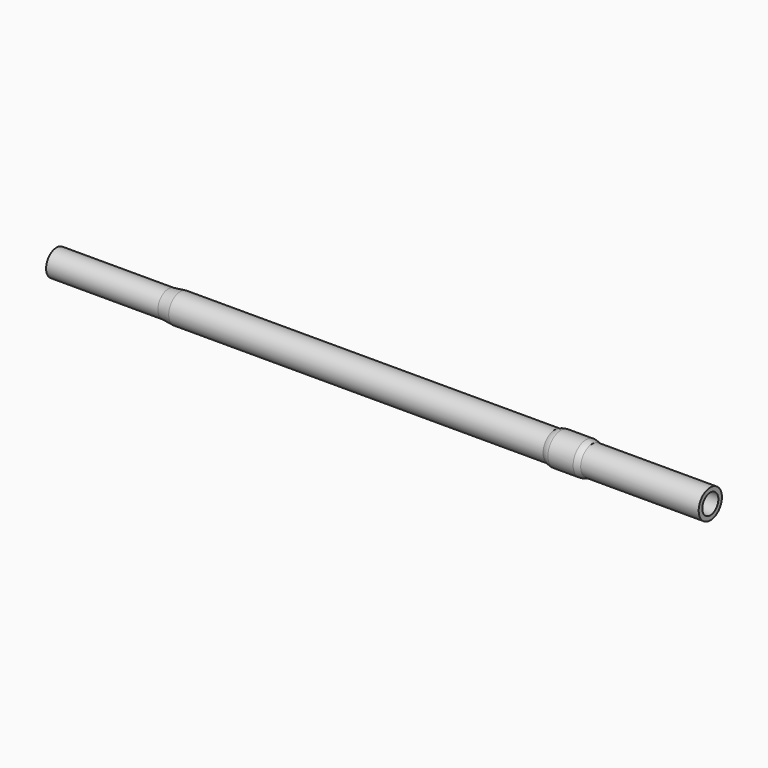
from build123d import *

# Parameters (mm, degrees)
F0_W = 5.08
F0_H = 0.5969
F3_D = 0.9144


# Not quite as in the source:
# - a fillet or chamfer that OpenCascade refuses, or shapes differently, is made with other operations: its cross-section is extruded or revolved along the edge and cut away or added


with BuildPart() as f1:
    # F0 (on Front) → F1 (revolve)
    with BuildSketch(Plane.XZ):
        with Locations((2.54, 0.29845)):
            Rectangle(F0_W, F0_H)
        Polygon((5.6251967326, 0.6604), (5.6251967326, 0), (29.718, 0), (29.718, 0.6604), (24.3530571461, 0.6604), (24.3530571461, 0.7366), (22.6445570588, 0.7366), (22.6431967326, 0.6604), align=None)
        Polygon((5.08, 0.5969), (5.08, 0), (5.6251967326, 0), (5.6251967326, 0.6604), align=None)
    revolve(axis=Axis((14.859, 0, 0), (1, 0, 0)))

    # F3 (through all)
    with Locations(Plane(origin=(0, 0, 0), x_dir=(0, 1, 0), z_dir=(-1, 0, 0))):
        with Locations((0, 0)):
            Hole(F3_D / 2)

    # F4: fillet of radius 0.5588 on 1 edges, made by hand

    # F4_s1 → F4_t2 (revolve, cut)
    with BuildSketch(Plane.XZ):
        with BuildLine():
            ThreePointArc((24.3530571461, 0.6604), (24.21726941, 0.7172137188), (24.0713575188, 0.7366))
            Line((24.0713575188, 0.7366), (24.3530571461, 0.7366))
            Line((24.3530571461, 0.7366), (24.3530571461, 0.6604))
        make_face()
    revolve(axis=Axis((24.3530571461, 0, 0), (1, 0, 0)), mode=Mode.SUBTRACT)

    # F5: fillet of radius 0.5588 on 1 edges, made by hand

    # F5_s1 → F5_t2 (revolve, cut)
    with BuildSketch(Plane.XZ):
        with BuildLine():
            ThreePointArc((22.6431967326, 0.6604), (22.7789844686, 0.7172137188), (22.9248963599, 0.7366))
            Line((22.9248963599, 0.7366), (22.6445570588, 0.7366))
            Line((22.6445570588, 0.7366), (22.6431967326, 0.6604))
        make_face()
    revolve(axis=Axis((22.6445570588, 0, 0), (1, 0, 0)), mode=Mode.SUBTRACT)


solid = f1.part
